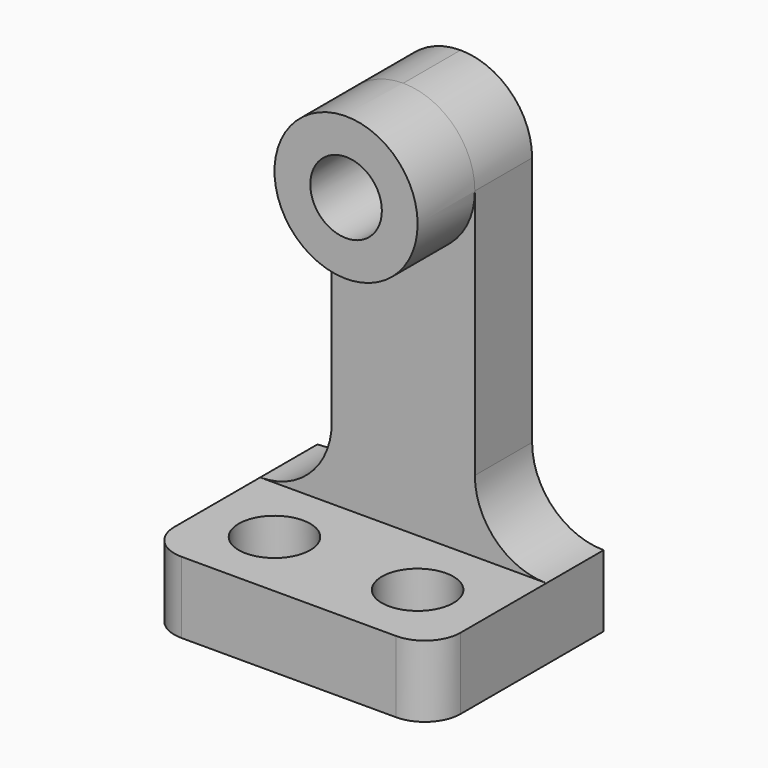
from build123d import *

# Parameters (mm, degrees)
F0_W      = 50.8
F0_H      = 38.1
F1_DEPTH  = 12.7
F2_R      = 6.35
F3_R      = 6.35
F4_DEPTH  = 25.4
F5_W      = 25.4
F5_H      = 12.7
F6_DEPTH  = 69.85
F7_R      = 12.69999
F8_W      = 12.7
F8_H      = 12.7
F9_DEPTH  = 12.7
F11_DEPTH = 25.4
F12_R     = 12.7
F13_DEPTH = 12.7
F14_R     = 6.35
F15_DEPTH = 25.4


# Not quite as in the source:
# - a fillet or chamfer is up to 0.001 mm smaller than in the source, because OpenCascade refuses the exact size


with BuildPart() as f1:
    # F0 (on Top) → F1 (new body)
    with BuildSketch(Plane.XY):
        with Locations((25.4, 19.05)):
            Rectangle(F0_W, F0_H)
    extrude(amount=F1_DEPTH)

    # F2
    f2_edges = [f1.edges().sort_by_distance(p)[0] for p in [
        (0, 0, 6.35),
        (50.8, 0, 6.35),
    ]]
    fillet(f2_edges, radius=F2_R)

    # F3 (on face) → F4 (cut)
    with BuildSketch(Plane.XY.offset(12.7)):
        with Locations((12.7, 12.7)):
            Circle(F3_R)
        with Locations((38.1, 12.7)):
            Circle(F3_R)
    extrude(amount=-F4_DEPTH, mode=Mode.SUBTRACT)

    # F5 (on face) → F6 (join)
    with BuildSketch(Plane.XY.offset(12.7)):
        with Locations((25.4, 31.75)):
            Rectangle(F5_W, F5_H)
    extrude(amount=F6_DEPTH)

    # F7 (radius 12.7 in the source; OpenCascade refuses exactly that, so slightly less here)
    f7_edges = [f1.edges().sort_by_distance(p)[0] for p in [
        (38.1, 31.75, 82.55),
        (12.7, 31.75, 82.55),
    ]]
    fillet(f7_edges, radius=F7_R)

    # F8 (on face) → F9 (join)
    with BuildSketch(Plane.XY.offset(12.7)):
        with Locations((6.35, 31.75)):
            Rectangle(F8_W, F8_H)
        with Locations((44.45, 31.75)):
            Rectangle(F8_W, F8_H)
    extrude(amount=F9_DEPTH)

    # F10 (on face) → F11 (cut)
    with BuildSketch(Plane.XZ.offset(-25.4)):
        with BuildLine():
            Line((0, 25.4), (0, 12.7))
            ThreePointArc((0, 12.7), (8.9802561211, 16.4197438789), (12.7, 25.4))
            Line((12.7, 25.4), (0, 25.4))
        make_face()
        with BuildLine():
            ThreePointArc((38.1, 25.4), (41.8197438789, 16.4197438789), (50.8, 12.7))
            Line((50.8, 12.7), (50.8, 25.4))
            Line((50.8, 25.4), (38.1, 25.4))
        make_face()
    extrude(amount=-F11_DEPTH, mode=Mode.SUBTRACT)

    # F12 (on face) → F13 (join)
    with BuildSketch(Plane.XZ.offset(-25.4)):
        with Locations((25.4, 69.85)):
            Circle(F12_R)
    extrude(amount=F13_DEPTH)

    # F14 (on face) → F15 (cut)
    with BuildSketch(Plane.XZ.offset(-12.7)):
        with Locations((25.4, 69.85)):
            Circle(F14_R)
    extrude(amount=-F15_DEPTH, mode=Mode.SUBTRACT)


solid = f1.part
